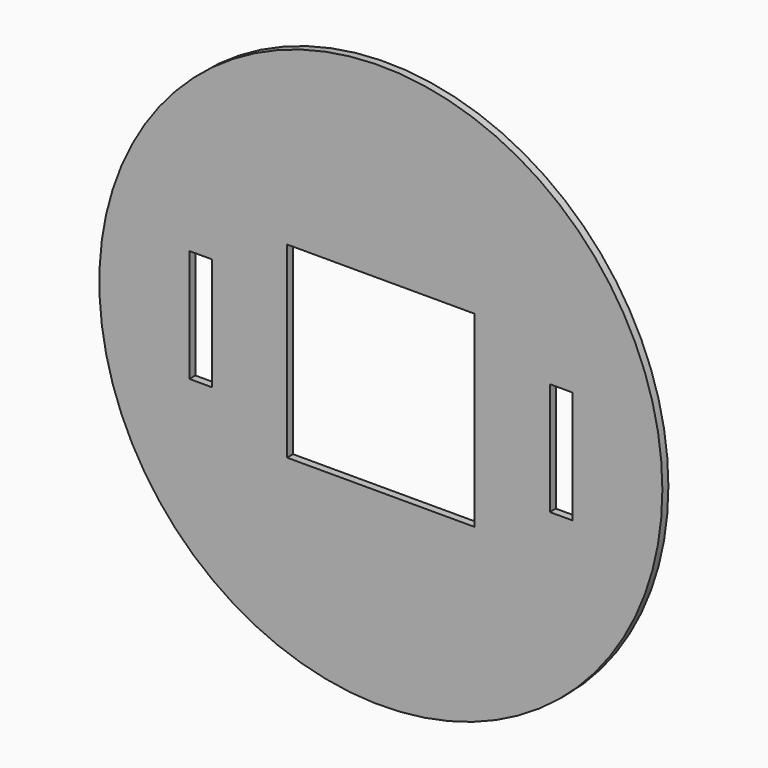
from build123d import *

# Parameters (mm, degrees)
F2_R     = 75
F2_W     = 50
F2_H     = 50
F3_DEPTH = 2


# Not quite as in the source:
# - a feature of the source that left no trace in its solid (it failed there, or was rolled back) is left out


with BuildPart() as f3:
    # F2 (on offset) → F3 (new body)
    with BuildSketch(Plane.XZ.offset(60)):
        Circle(F2_R)
        Polygon((-45, 15), (-45, 0), (-45, -15), (-51, -15), (-51, 15), align=None, mode=Mode.SUBTRACT)
        Rectangle(F2_W, F2_H, mode=Mode.SUBTRACT)
        Polygon((45, -15), (45, 0), (45, 15), (51, 15), (51, -15), align=None, mode=Mode.SUBTRACT)
    extrude(amount=F3_DEPTH)


solid = f3.part
